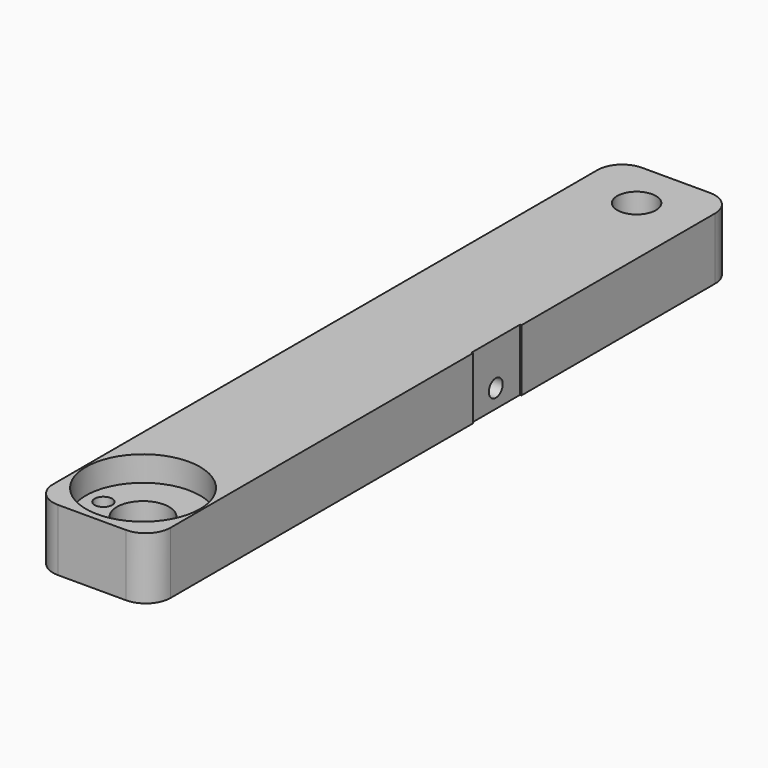
from build123d import *

# Parameters (mm, degrees)
F0_W      = 24.13
F0_H      = 149.86
F1_DEPTH  = 12.7
F2_W      = 12.446
F2_H      = 20.32
F3_DEPTH  = 0.29765625
F4_R      = 3.96875
F5_DEPTH  = 25.4
F7_R      = 1.7859375
F8_DEPTH  = 25.4
F6_R      = 11.7078125
F9_DEPTH  = 5.159375
F10_R     = 5.3578125
F11_DEPTH = 25.4
F12_R     = 1.7907
F13_DEPTH = 25.4
F14_R     = 5.08
F16_DEPTH = 2.778125


# Not quite as in the source:
# - a length typed as a fraction of an inch, garbled in the dataset ("3 / 203.2 mm" for 3/8 in), is restored


with BuildPart() as f1:
    # F0 (on Top) → F1 (new body)
    with BuildSketch(Plane.XY):
        with Locations((0, -13.97)):
            Rectangle(F0_W, F0_H)
    extrude(amount=F1_DEPTH)

    # F2 (on face) → F3 (cut)
    with BuildSketch(Plane.YZ.offset(12.065)):
        with Locations((0, 2.54)):
            Rectangle(F2_W, F2_H)
    extrude(amount=-F3_DEPTH, mode=Mode.SUBTRACT)

    # F4 (on face) → F5 (cut)
    with BuildSketch(Plane.XY.offset(12.7)):
        with Locations((0, 50.8381508)):
            Circle(F4_R)
    extrude(amount=-F5_DEPTH, mode=Mode.SUBTRACT)

    # F7 (on face) → F8 (cut)
    with BuildSketch(Plane.YZ.offset(11.76734375)):
        with Locations((0, 3.7703125)):
            Circle(F7_R)
    extrude(amount=-F8_DEPTH, mode=Mode.SUBTRACT)

    # F6 (on face) → F9 (cut)
    with BuildSketch(Plane.XY.offset(12.7)):
        with Locations((0, -75.803125)):
            Circle(F6_R)
    extrude(amount=-F9_DEPTH, mode=Mode.SUBTRACT)

    # F10 (on face) → F11 (cut)
    with BuildSketch(Plane.XY.offset(7.540625)):
        with Locations((0, -75.803125)):
            Circle(F10_R)
    extrude(amount=-F11_DEPTH, mode=Mode.SUBTRACT)

    # F12 (on face) → F13 (cut)
    with BuildSketch(Plane.XY.offset(7.540625)):
        with Locations((-8.1359375, -75.803125)):
            Circle(F12_R)
        with Locations((8.1359375, -75.803125)):
            Circle(F12_R)
    extrude(amount=-F13_DEPTH, mode=Mode.SUBTRACT)

    # F14
    f14_edges = [f1.edges().sort_by_distance(p)[0] for p in [
        (-12.065, -88.9, 6.35),
        (12.065, -88.9, 6.35),
        (-12.065, 60.96, 6.35),
        (12.065, 60.96, 6.35),
    ]]
    fillet(f14_edges, radius=F14_R)

    # F15 (on face) → F16 (cut)
    with BuildSketch(Plane(origin=(-12.065, 0, 0), x_dir=(0, -1, 0), z_dir=(-1, 0, 0))):
        Polygon((2.2913588808, 7.7390625), (-2.2913588808, 7.7390625), (-4.5827177617, 3.7703125), (-2.2913588808, -0.1984375), (2.2913588808, -0.1984375), (4.5827177617, 3.7703125), align=None)
    extrude(amount=-F16_DEPTH, mode=Mode.SUBTRACT)


solid = f1.part
